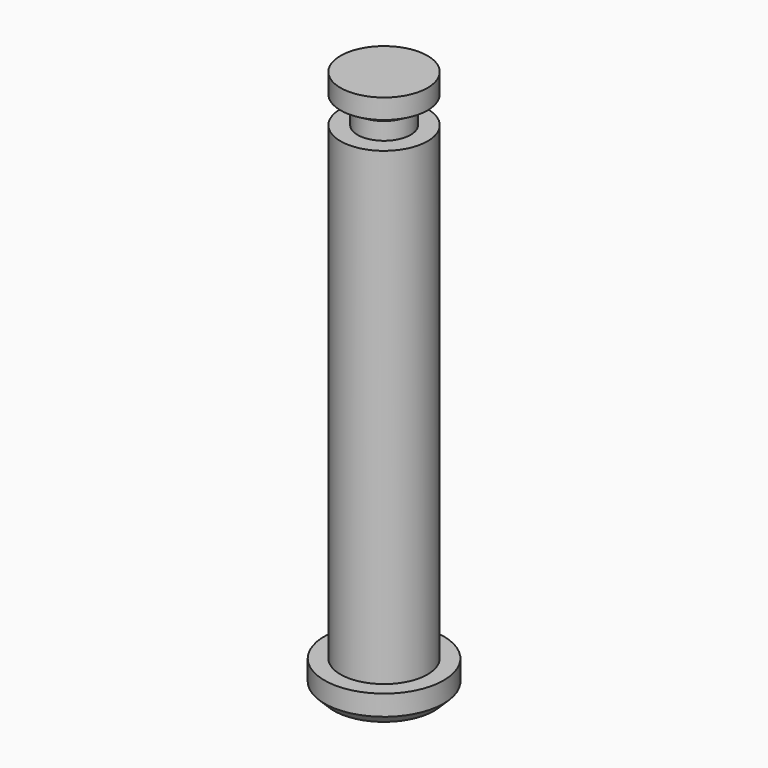
from build123d import *

# Parameters (mm, degrees)
F0_R     = 6.35
F1_DEPTH = 3.175
F2_R     = 4.6355
F3_DEPTH = 55
F6_SIZE  = 1


# Not quite as in the source:
# - a length typed as a fraction of an inch, garbled in the dataset ("3 / 203.2 mm" for 3/8 in), is restored


with BuildPart() as f1:
    # F0 (on Top) → F1 (new body)
    with BuildSketch(Plane.XY):
        Circle(F0_R)
    extrude(amount=F1_DEPTH)

    # F2 (on face) → F3 (join)
    with BuildSketch(Plane.XY.offset(3.175)):
        Circle(F2_R)
    extrude(amount=F3_DEPTH)

    # F4 (on Right) → F5 (revolve, cut)
    with BuildSketch(Plane.YZ):
        Polygon((-2.8230392858, 55.0202994616), (-4.8230392858, 56.175), (-4.8230392858, 53.175), (-2.8230392858, 53.175), align=None)
    revolve(axis=Axis((0, 0, 58.175), (0, 0, 1)), mode=Mode.SUBTRACT)

    # F6
    f6_edges = [f1.edges().sort_by_distance(p)[0] for p in [
        (-6.35, 0, 0),
    ]]
    chamfer(f6_edges, length=F6_SIZE)


solid = f1.part
